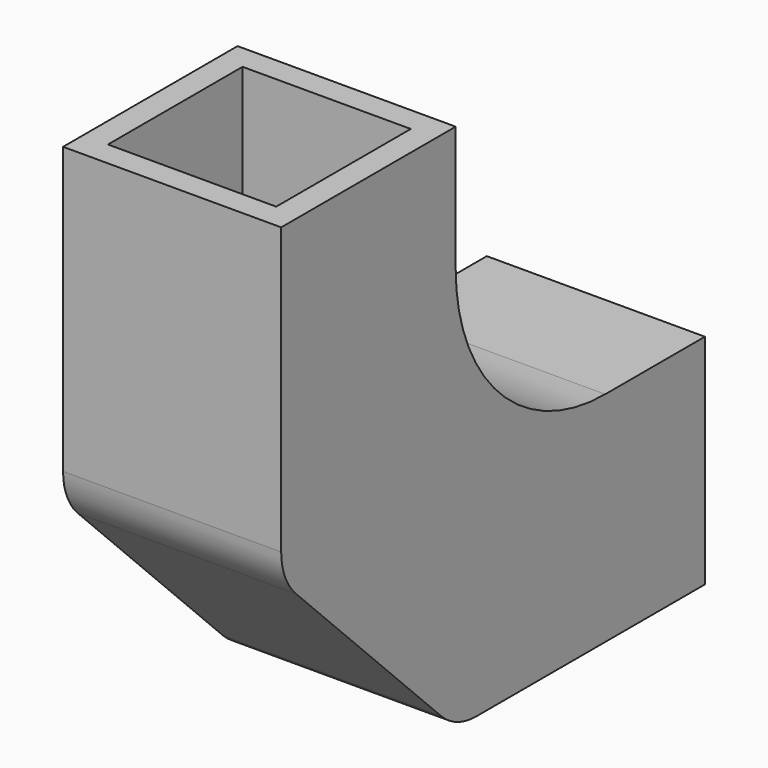
from build123d import *

# Parameters (mm, degrees)
F1_W        = 17.5
F1_H        = 17.5
F1_W_2      = 13.5
F1_H_2      = 13.5
F2_DEPTH    = 25
F3_W        = 17.5
F3_H        = 17.5
F3_W_2      = 13.5
F3_H_2      = 13.5
F4_DEPTH    = 25
F6_DEPTH    = 17.5
F7_T1_DEPTH = 18.2385988642
F7_T3_DEPTH = 27.8540843944
F7_T5_DEPTH = 27.867199163
F8_R        = 15


# Not quite as in the source:
# - a fillet or chamfer that OpenCascade refuses, or shapes differently, is made with other operations: its cross-section is extruded or revolved along the edge and cut away or added


with BuildPart() as f2:
    # F1 (on Top) → F2 (new body)
    with BuildSketch(Plane.XY):
        Rectangle(F1_W, F1_H)
        Rectangle(F1_W_2, F1_H_2, mode=Mode.SUBTRACT)
    extrude(amount=F2_DEPTH)

    # F3 (on face) → F4 (join)
    with BuildSketch(Plane(origin=(0, 8.75, 0), x_dir=(-1, 0, 0), z_dir=(0, 1, 0))):
        with Locations((0, -8.75)):
            Rectangle(F3_W, F3_H)
        with Locations((0, -8.75)):
            Rectangle(F3_W_2, F3_H_2, mode=Mode.SUBTRACT)
    extrude(amount=F4_DEPTH)

    # F5 (on face) → F6 (join, through all)
    with BuildSketch(Plane(origin=(-8.75, 0, 0), x_dir=(0, -1, 0), z_dir=(-1, 0, 0))):
        Polygon((-8.75, 0), (-8.75, -17.5), (8.7529988959, 0), align=None)
    extrude(amount=-F6_DEPTH)

    # F7: fillet of radius 5 on 3 edges, made by hand

    # F7_s2 → F7_t1 (cut)
    with BuildSketch(Plane.YZ.offset(-9.1192994321)):
        with BuildLine():
            ThreePointArc((-8.75, 0), (-8.6996483838, -0.052591736), (-8.6485362941, -0.1044447036))
            Line((-8.6485362941, -0.1044447036), (-8.7529988959, 0))
            Line((-8.7529988959, 0), (-8.75, 0))
        make_face()
    extrude(amount=F7_T1_DEPTH, mode=Mode.SUBTRACT)

    # F7_s4 → F7_t3 (cut)
    with BuildSketch(Plane.YZ.offset(-13.9270421972)):
        with BuildLine():
            ThreePointArc((7.2855858942, -16.0358368012), (8.9075976032, -17.1194796247), (10.8208168789, -17.5))
            Line((10.8208168789, -17.5), (8.75, -17.5))
            Line((8.75, -17.5), (7.2855858942, -16.0358368012))
        make_face()
    extrude(amount=F7_T3_DEPTH, mode=Mode.SUBTRACT)

    # F7_s6 → F7_t5 (cut)
    with BuildSketch(Plane.YZ.offset(-13.9335995815)):
        with BuildLine():
            ThreePointArc((-8.75, 2.0683203716), (-8.3693156919, 0.1547053272), (-7.2852309847, -1.4675164296))
            Line((-7.2852309847, -1.4675164296), (-7.6387540831, -1.8211001097))
            ThreePointArc((-7.6387540831, -1.8211001097), (-9.0020593926, -0.4580283837), (-9.1136694691, -0.3431392098))
            Line((-9.1136694691, -0.3431392098), (-9.25, 0))
            Line((-9.25, 0), (-9.25, 2.0683203716))
            Line((-9.25, 2.0683203716), (-8.75, 2.0683203716))
        make_face()
    extrude(amount=F7_T5_DEPTH, mode=Mode.SUBTRACT)

    # F8
    f8_edges = [f2.edges().sort_by_distance(p)[0] for p in [
        (0, 8.75, 0),
    ]]
    fillet(f8_edges, radius=F8_R)


solid = f2.part
